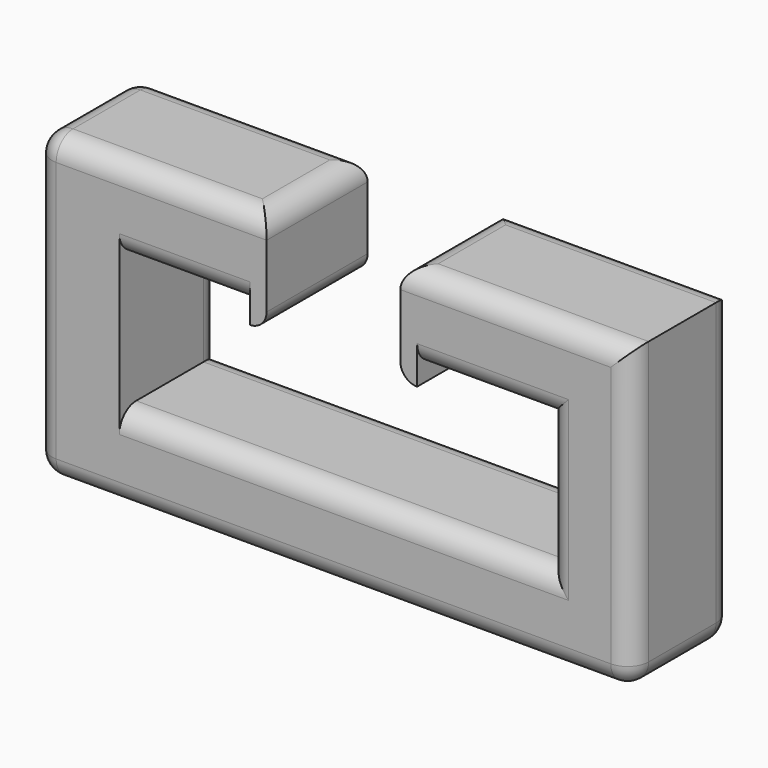
from build123d import *

# Parameters (mm, degrees)
F1_DEPTH = 3
F2_R     = 0.5
F3_R     = 0.39999


# Not quite as in the source:
# - a fillet or chamfer is up to 0.001 mm smaller than in the source, because OpenCascade refuses the exact size


with BuildPart() as f1:
    # F0 (on Front) → F1 (new body)
    with BuildSketch(Plane.XZ):
        Polygon((-7.0882368928, 3.6), (-7.0882368928, -3.6), (7.0882368928, -3.6), (7.0882368928, 3.6), (1.5882368928, 3.6), (1.5882368928, 1.6), (1.5882368928, 1.2), (1.9882368928, 1.2), (1.9882368928, 1.6), (5.0882368928, 1.6), (5.0882368928, -1.6), (-5.0882368928, -1.6), (-5.0882368928, 1.6), (-1.9882368928, 1.6), (-1.9882368928, 1.2), (-1.5882368928, 1.2), (-1.5882368928, 1.6), (-1.5882368928, 3.6), align=None)
    extrude(amount=F1_DEPTH)

    # F2
    f2_edges = [f1.edges().sort_by_distance(p)[0] for p in [
        (4.338237, 0, 3.6),
        (-4.338237, 0, 3.6),
        (-7.088237, 0, 0),
        (0, 0, -3.6),
        (7.088237, 0, 0),
        (1.588237, -1.5, 3.6),
        (-1.588237, -1.5, 3.6),
        (-4.338237, -3, 3.6),
        (-7.088237, -1.5, 3.6),
        (4.338237, -3, 3.6),
        (3.538237, -3, 1.6),
        (-3.538237, -3, 1.6),
        (3.538237, 0, 1.6),
        (-3.538237, 0, 1.6),
        (-7.088237, -3, 0),
        (7.088237, -3, 0),
        (5.088237, -3, 0),
        (-5.088237, 0, 0),
        (-7.088237, -1.5, -3.6),
        (7.088237, -1.5, -3.6),
        (5.088237, 0, 0),
        (0, 0, -1.6),
        (0, -3, -1.6),
        (0, -3, -3.6),
    ]]
    fillet(f2_edges, radius=F2_R)

    # F3 (radius 0.4 in the source; OpenCascade refuses exactly that, so slightly less here)
    f3_edges = [f1.edges().sort_by_distance(p)[0] for p in [
        (1.588237, -1.5, 1.2),
        (-1.588237, -1.5, 1.2),
    ]]
    fillet(f3_edges, radius=F3_R)


solid = f1.part
